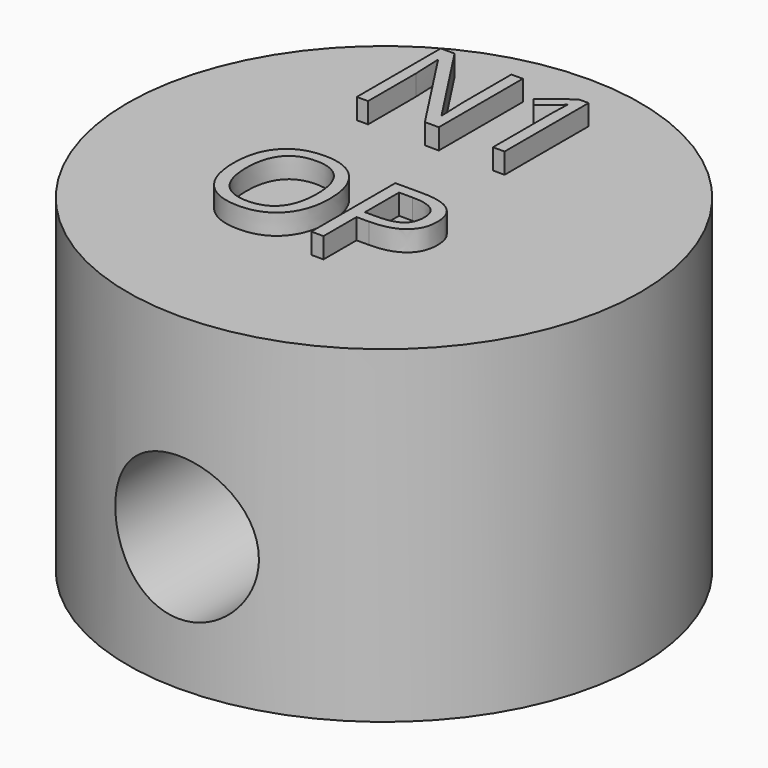
from build123d import *

# Parameters (mm, degrees)
F0_R         = 12.5
F1_DEPTH     = 16
F3_R         = 3.5
F4_DEPTH     = 25.001
F5_TEXT_SIZE = 7.171671896
F6_DEPTH     = 1


# Not quite as in the source:
# - Text() gives the source's letters only with a copy of the font that has no kerning and outlines rounded to 1/6400 em; it was checked with that copy


with BuildPart() as f1:
    # F0 (on Top) → F1 (new body)
    with BuildSketch(Plane.XY):
        Circle(F0_R)
    extrude(amount=F1_DEPTH)

    # F3 (on offset) → F4 (cut, through all)
    with BuildSketch(Plane.XZ.offset(-12.5)):
        with Locations((0, 6.5)):
            Circle(F3_R)
    extrude(amount=F4_DEPTH, mode=Mode.SUBTRACT)

    # F5 (on face) → F6 (join)
    with BuildSketch(Plane.XY.offset(16)):
        with Locations((-5.5, 4.3363962349)):
            Text('N1', F5_TEXT_SIZE, font='Open Sans', text_align=(TextAlign.LEFT, TextAlign.BOTTOM))
        with Locations((-5.5, -5.4170775437)):
            Text('OP', F5_TEXT_SIZE, font='Open Sans', text_align=(TextAlign.LEFT, TextAlign.BOTTOM))
    extrude(amount=F6_DEPTH)


solid = f1.part
